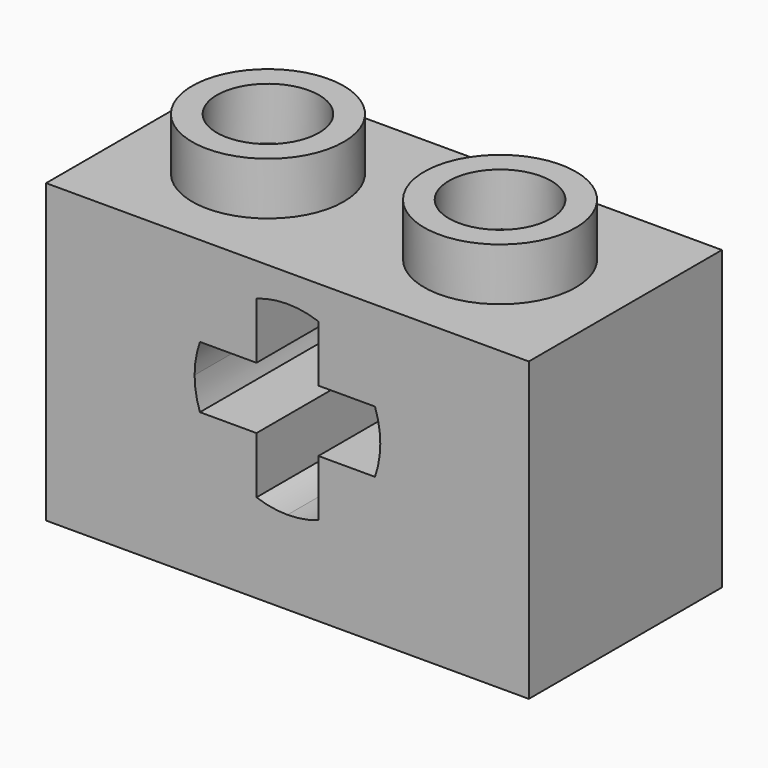
from build123d import *

# Parameters (mm, degrees)
F0_W     = 15.6
F0_H     = 9.6
F1_DEPTH = 7.8
F2_R     = 2.45
F2_R_2   = 1.65
F3_DEPTH = 1.7
F5_DEPTH = 2


# Not quite as in the source:
# - a feature names something its author has since deleted; it is built from what else it names


with BuildPart() as f1:
    # F0 (on Front) → F1 (new body)
    with BuildSketch(Plane.XZ):
        with Locations((7.5497636572, 4.7150965011)):
            Rectangle(F0_W, F0_H)
        with BuildLine():
            Line((10.5497636572, 6.6150965011), (10.5497636572, 5.6150965011))
            Line((10.5497636572, 5.6150965011), (10.5497636572, 4.6150965011))
            Line((10.5497636572, 4.6150965011), (10.3781907819, 4.6150965011))
            ThreePointArc((10.3781907819, 4.6150965011), (9.6710840007, 3.4937761575), (8.5497636572, 2.7866693764))
            Line((8.5497636572, 2.7866693764), (8.5497636572, 2.6150965011))
            Line((8.5497636572, 2.6150965011), (7.5497636572, 2.6150965011))
            Line((7.5497636572, 2.6150965011), (6.5497636572, 2.6150965011))
            Line((6.5497636572, 2.6150965011), (6.5497636572, 2.7866693764))
            ThreePointArc((6.5497636572, 2.7866693764), (5.4284433136, 3.4937761575), (4.7213365324, 4.6150965011))
            Line((4.7213365324, 4.6150965011), (4.5497636572, 4.6150965011))
            Line((4.5497636572, 4.6150965011), (4.5497636572, 5.6150965067))
            Line((4.5497636572, 5.6150965067), (4.5497636572, 6.6150965011))
            Line((4.5497636572, 6.6150965011), (4.7213365324, 6.6150965011))
            ThreePointArc((4.7213365324, 6.6150965011), (5.4284433136, 7.7364168447), (6.5497636572, 8.4435236258))
            Line((6.5497636572, 8.4435236258), (6.5497636572, 8.6150965011))
            Line((6.5497636572, 8.6150965011), (7.5497636572, 8.6150965011))
            Line((7.5497636572, 8.6150965011), (8.5497636572, 8.6150965011))
            Line((8.5497636572, 8.6150965011), (8.5497636572, 8.4435236258))
            ThreePointArc((8.5497636572, 8.4435236258), (9.6710840007, 7.7364168447), (10.3781907819, 6.6150965011))
            Line((10.3781907819, 6.6150965011), (10.5497636572, 6.6150965011))
        make_face(mode=Mode.SUBTRACT)
        with BuildLine():
            ThreePointArc((8.5497636572, 2.7866693764), (9.6710840007, 3.4937761575), (10.3781907819, 4.6150965011))
            Line((10.3781907819, 4.6150965011), (8.5497636572, 4.6150965011))
            Line((8.5497636572, 4.6150965011), (8.5497636572, 2.7866693764))
        make_face()
        with BuildLine():
            Line((8.5497636572, 6.6150965011), (10.3781907819, 6.6150965011))
            ThreePointArc((10.3781907819, 6.6150965011), (9.6710840007, 7.7364168447), (8.5497636572, 8.4435236258))
            Line((8.5497636572, 8.4435236258), (8.5497636572, 6.6150965011))
        make_face()
        with BuildLine():
            Line((4.7213365324, 6.6150965011), (6.5497636572, 6.6150965011))
            Line((6.5497636572, 6.6150965011), (6.5497636572, 8.4435236258))
            ThreePointArc((6.5497636572, 8.4435236258), (5.4284433136, 7.7364168447), (4.7213365324, 6.6150965011))
        make_face()
        with BuildLine():
            Line((6.5497636572, 2.7866693764), (6.5497636572, 4.6150965011))
            Line((6.5497636572, 4.6150965011), (4.7213365324, 4.6150965011))
            ThreePointArc((4.7213365324, 4.6150965011), (5.4284433136, 3.4937761575), (6.5497636572, 2.7866693764))
        make_face()
        with BuildLine():
            Line((10.5497636572, 4.6150965011), (10.5497636572, 5.6150965011))
            ThreePointArc((10.5497636572, 5.6150965011), (10.5065593361, 5.1077905649), (10.3781907819, 4.6150965011))
            Line((10.3781907819, 4.6150965011), (10.5497636572, 4.6150965011))
        make_face()
        with BuildLine():
            ThreePointArc((10.3781907819, 6.6150965011), (10.5065593361, 6.1224024373), (10.5497636572, 5.6150965011))
            Line((10.5497636572, 5.6150965011), (10.5497636572, 6.6150965011))
            Line((10.5497636572, 6.6150965011), (10.3781907819, 6.6150965011))
        make_face()
        with BuildLine():
            ThreePointArc((7.5497636572, 8.6150965011), (8.0570695933, 8.5718921801), (8.5497636572, 8.4435236258))
            Line((8.5497636572, 8.4435236258), (8.5497636572, 8.6150965011))
            Line((8.5497636572, 8.6150965011), (7.5497636572, 8.6150965011))
        make_face()
        with BuildLine():
            ThreePointArc((6.5497636572, 8.4435236258), (7.042457721, 8.5718921801), (7.5497636572, 8.6150965011))
            Line((7.5497636572, 8.6150965011), (6.5497636572, 8.6150965011))
            Line((6.5497636572, 8.6150965011), (6.5497636572, 8.4435236258))
        make_face()
        with BuildLine():
            ThreePointArc((4.5497636572, 5.6150965067), (4.5929679787, 6.12240244), (4.7213365324, 6.6150965011))
            Line((4.7213365324, 6.6150965011), (4.5497636572, 6.6150965011))
            Line((4.5497636572, 6.6150965011), (4.5497636572, 5.6150965067))
        make_face()
        with BuildLine():
            Line((4.5497636572, 4.6150965011), (4.7213365324, 4.6150965011))
            ThreePointArc((4.7213365324, 4.6150965011), (4.5929679777, 5.1077905677), (4.5497636572, 5.6150965067))
            Line((4.5497636572, 5.6150965067), (4.5497636572, 4.6150965011))
        make_face()
        with BuildLine():
            Line((6.5497636572, 2.6150965011), (7.5497636572, 2.6150965011))
            ThreePointArc((7.5497636572, 2.6150965011), (7.042457721, 2.6583008221), (6.5497636572, 2.7866693764))
            Line((6.5497636572, 2.7866693764), (6.5497636572, 2.6150965011))
        make_face()
        with BuildLine():
            Line((8.5497636572, 2.6150965011), (8.5497636572, 2.7866693764))
            ThreePointArc((8.5497636572, 2.7866693764), (8.0570695933, 2.6583008221), (7.5497636572, 2.6150965011))
            Line((7.5497636572, 2.6150965011), (8.5497636572, 2.6150965011))
        make_face()
    extrude(amount=F1_DEPTH)

    # F2 (on face) → F3 (join)
    with BuildSketch(Plane.XY.offset(9.5150965011)):
        with Locations((3.7997636572, -3.9)):
            Circle(F2_R)
        with Locations((3.7997636572, -3.9)):
            Circle(F2_R_2, mode=Mode.SUBTRACT)
        with Locations((11.2997636572, -3.9)):
            Circle(F2_R)
        with Locations((11.2997636572, -3.9)):
            Circle(F2_R_2, mode=Mode.SUBTRACT)
    extrude(amount=F3_DEPTH)

    # F4 (on face) → F5 (cut)
    with BuildSketch(Plane(origin=(0, 0, -0.0849034989), x_dir=(1, 0, 0), z_dir=(0, 0, -1))):
        Polygon((1.3497636572, 6.2), (1.3497636572, 3.9), (1.3497636572, 1.6), (7.5497636572, 1.6), (13.7497636572, 1.6), (13.7497636572, 3.9), (13.7497636572, 6.2), (7.5497636572, 6.2), align=None)
    extrude(amount=-F5_DEPTH, mode=Mode.SUBTRACT)


solid = f1.part
